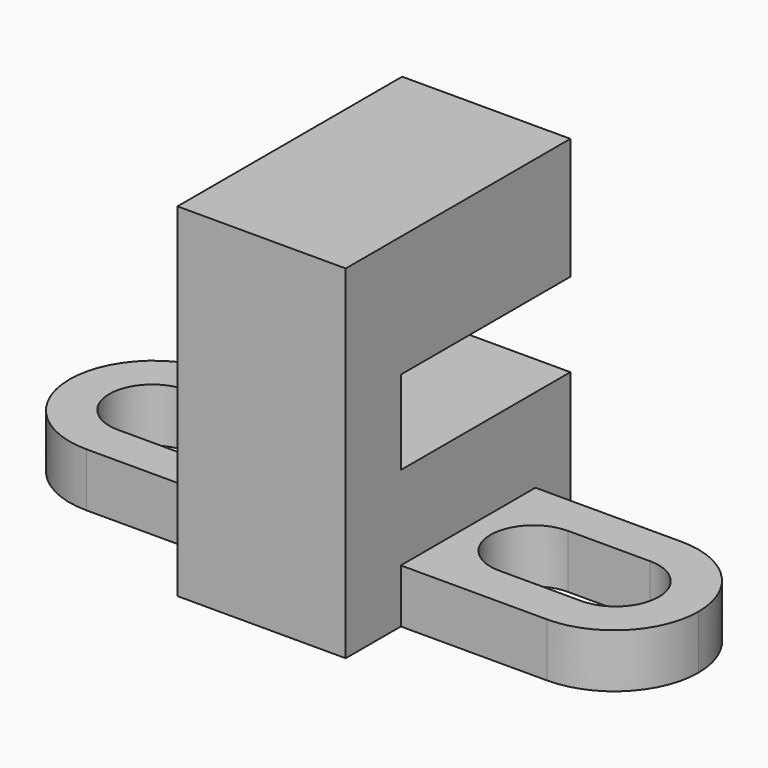
from build123d import *

# Parameters (mm, degrees)
F0_W     = 10.6
F0_H     = 12.954
F1_DEPTH = 6.35
F2_W     = 8
F2_H     = 3.17
F3_DEPTH = 6.351
F4_W     = 6.35
F4_H     = 2.03
F5_DEPTH = 8.695
F6_R     = 3.17499
F9_DEPTH = 2.031


# Not quite as in the source:
# - a fillet or chamfer is up to 0.001 mm smaller than in the source, because OpenCascade refuses the exact size
# - a pattern or mirror of a feature is missing from the dataset's text; its kind, count and spacing are read off the source's solid


with BuildPart() as f1:
    # F0 (on Right) → F1 (new body)
    with BuildSketch(Plane.YZ):
        with Locations((5.3, 6.477)):
            Rectangle(F0_W, F0_H)
    extrude(amount=-F1_DEPTH)

    # F2 (on face) → F3 (cut, through all)
    with BuildSketch(Plane.YZ):
        with Locations((6.6, 6.785)):
            Rectangle(F2_W, F2_H)
    extrude(amount=-F3_DEPTH, mode=Mode.SUBTRACT)

    # F4 (on face) → F5 (join)
    with BuildSketch(Plane.YZ):
        with Locations((5.775, 1.015)):
            Rectangle(F4_W, F4_H)
    f5 = extrude(amount=F5_DEPTH)

    # F5_copies: F5 across plane
    add(f5.mirror(Plane(origin=(-3.174997, 0, 0), x_dir=(0, 0, -1), z_dir=(-1, 0, 0))))

    # F6 (radius 3.175 in the source; OpenCascade refuses exactly that, so slightly less here)
    f6_edges = [f1.edges().sort_by_distance(p)[0] for p in [
        (8.695, 2.6, 1.015),
        (8.695, 8.95, 1.015),
        (-15.044994, 8.95, 1.015),
        (-15.044994, 2.6, 1.015),
    ]]
    fillet(f6_edges, radius=F6_R)

    # F8 (on face) → F9 (cut, through all)
    with BuildSketch(Plane.XY.offset(2.03)):
        with BuildLine():
            Line((2.47, 4.15), (5.57, 4.15))
            ThreePointArc((5.57, 4.15), (7.195, 5.775), (5.57, 7.4))
            Line((5.57, 7.4), (2.47, 7.4))
            ThreePointArc((2.47, 7.4), (0.845, 5.775), (2.47, 4.15))
        make_face()
    f9 = extrude(amount=-F9_DEPTH, mode=Mode.SUBTRACT)

    # F9_copies: F9 across plane
    add(f9.mirror(Plane(origin=(-3.175, 0, 0), x_dir=(0, 0, -1), z_dir=(-1, 0, 0))), mode=Mode.SUBTRACT)


solid = f1.part
